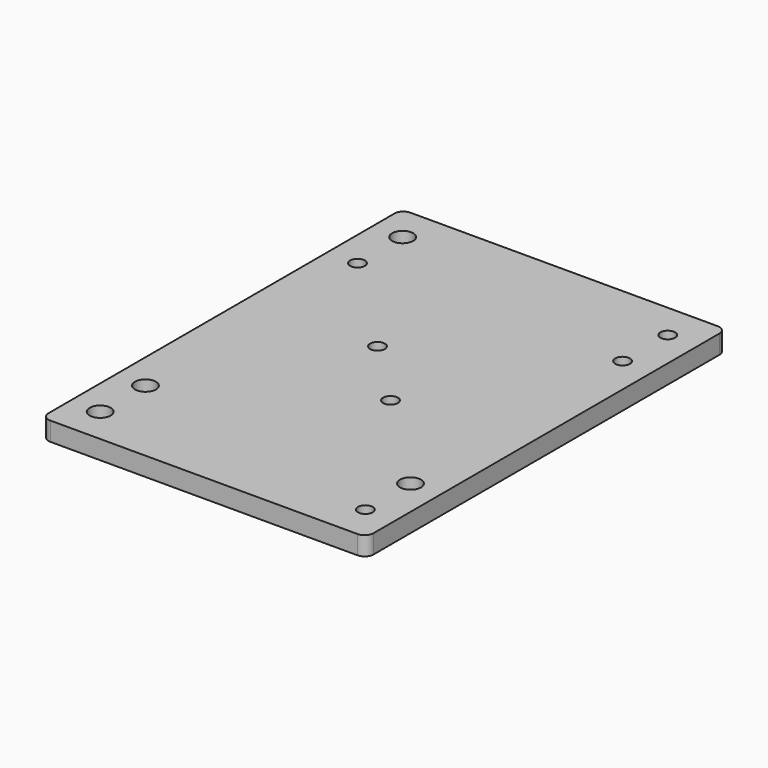
from build123d import *

# Parameters (mm, degrees)
F0_R     = 3.56
F0_R_2   = 2.5
F1_DEPTH = 6.35


# Not quite as in the source:
# - a length typed as a fraction of an inch, garbled in the dataset ("3 / 203.2 mm" for 3/8 in), is restored


with BuildPart() as f1:
    # F0 (on Top) → F1 (new body)
    with BuildSketch(Plane.XY):
        with BuildLine():
            ThreePointArc((55, 73.2), (54.1213203436, 75.3213203436), (52, 76.2))
            Line((52, 76.2), (-52, 76.2))
            ThreePointArc((-52, 76.2), (-54.1213203436, 75.3213203436), (-55, 73.2))
            Line((-55, 73.2), (-55, -73.2))
            ThreePointArc((-55, -73.2), (-54.1213203436, -75.3213203436), (-52, -76.2))
            Line((-52, -76.2), (52, -76.2))
            ThreePointArc((52, -76.2), (54.1213203436, -75.3213203436), (55, -73.2))
            Line((55, -73.2), (55, 73.2))
        make_face()
        with Locations((-44.875, -64)):
            Circle(F0_R, mode=Mode.SUBTRACT)
        with Locations((-44.875, -44.875)):
            Circle(F0_R, mode=Mode.SUBTRACT)
        with Locations((44.875, -64)):
            Circle(F0_R_2, mode=Mode.SUBTRACT)
        with Locations((44.875, -44.875)):
            Circle(F0_R, mode=Mode.SUBTRACT)
        with Locations((11, -11)):
            Circle(F0_R_2, mode=Mode.SUBTRACT)
        with Locations((-11, 11)):
            Circle(F0_R_2, mode=Mode.SUBTRACT)
        with Locations((-44.875, 44.875)):
            Circle(F0_R_2, mode=Mode.SUBTRACT)
        with Locations((-44.875, 64)):
            Circle(F0_R, mode=Mode.SUBTRACT)
        with Locations((44.875, 44.875)):
            Circle(F0_R_2, mode=Mode.SUBTRACT)
        with Locations((44.875, 64)):
            Circle(F0_R_2, mode=Mode.SUBTRACT)
    extrude(amount=F1_DEPTH)


solid = f1.part
